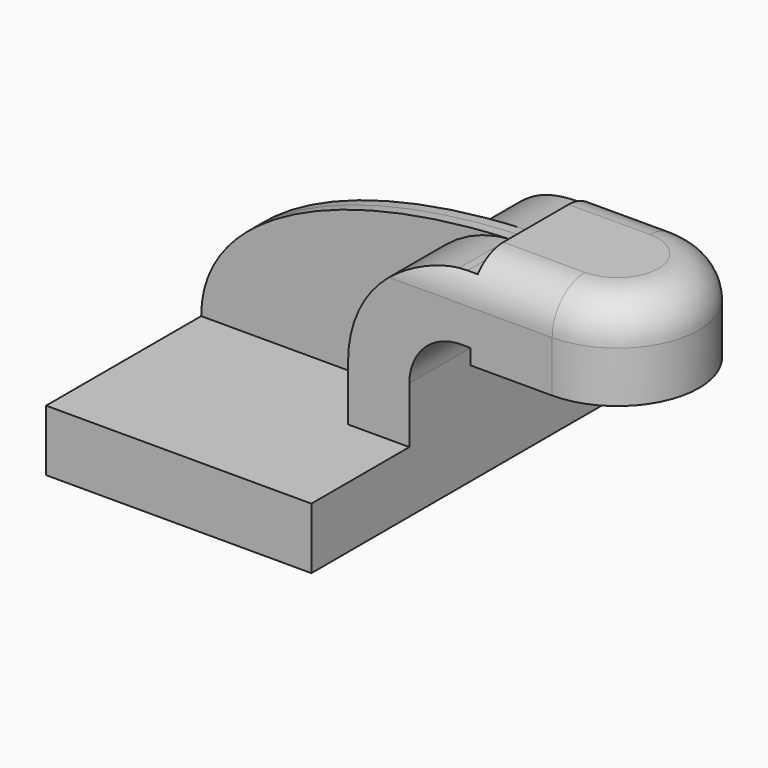
from build123d import *

# Parameters (mm, degrees)
F1_DEPTH = 63.5
F0_W     = 25.4
F0_H     = 19.05
F0_H_2   = 4.7498
F0_H_3   = 4.7752
F2_DEPTH = 25.4
F4_DEPTH = 3.175
F5_R     = 12.7


with BuildPart() as f1:
    # F0 (on Front) → F1 (new body, symmetric)
    with BuildSketch(Plane.XZ):
        Polygon((-41.275, -9.525), (41.275, -9.525), (41.275, 9.525), (22.225, 9.525), (-41.275, 9.525), align=None)
    extrude(amount=F1_DEPTH, both=True)

    # F0 (on Front) → F2 (join, symmetric)
    with BuildSketch(Plane.XZ):
        with BuildLine():
            Line((22.225, 9.525), (41.275, 9.525))
            Line((41.275, 9.525), (41.275, 27.0002))
            ThreePointArc((41.275, 27.0002), (45.9246798487, 38.2255201513), (57.15, 42.8752))
            Line((57.15, 42.8752), (60.325, 42.8752))
            Line((60.325, 42.8752), (60.325, 61.9252))
            Line((60.325, 61.9252), (57.15, 61.9252))
            add(Edge.make_bspline(
                [(54.6251217416, 61.8338132892), (55.4640803854, 61.8685780106), (56.3057470428, 61.8990488271), (57.15, 61.9252)],
                knots=[109.7820212307, 109.7820212307, 109.7820212307, 109.7820212307, 111.5045361635, 111.5045361635, 111.5045361635, 111.5045361635], degree=3))
            ThreePointArc((54.6251217416, 61.8338132892), (31.5771921939, 50.7864802033), (22.225, 27.0002))
            Line((22.225, 27.0002), (22.225, 9.525))
        make_face()
        with Locations((73.025, 52.4002)):
            Rectangle(F0_W, F0_H)
        with Locations((73.025, 64.3001)):
            Rectangle(F0_W, F0_H_2)
        with Locations((73.025, 40.4876)):
            Rectangle(F0_W, F0_H_3)
    extrude(amount=F2_DEPTH, both=True)

    # F0 (on Front) → F3 (revolve)
    with BuildSketch(Plane.XZ):
        Polygon((85.725, 61.9252), (85.725, 42.8752), (85.725, 38.1), (111.125, 38.1), (111.125, 66.675), (85.725, 66.675), align=None)
    revolve(axis=Axis((85.725, 0, 52.3875), (0, 0, 1)))

    # F0 (on Front) → F4 (join, symmetric)
    with BuildSketch(Plane.XZ):
        with BuildLine():
            add(Edge.make_bspline(
                [(-41.275, 9.525), (-41.3146686629, 39.9607514864), (1.1552946366, 59.618133583), (54.6251217416, 61.8338132892)],
                knots=[0, 0, 0, 0, 109.7820212307, 109.7820212307, 109.7820212307, 109.7820212307], degree=3))
            Line((-41.275, 9.525), (22.225, 9.525))
            Line((22.225, 9.525), (22.225, 27.0002))
            ThreePointArc((22.225, 27.0002), (31.5771921939, 50.7864802033), (54.6251217416, 61.8338132892))
        make_face()
    extrude(amount=F4_DEPTH, both=True)

    # F5
    f5_edges = [f1.edges().sort_by_distance(p)[0] for p in [
        (85.725, 25.4, 52.3875),
        (73.025, 25.4, 66.675),
        (73.025, -25.4, 66.675),
        (111.125, 0, 66.675),
    ]]
    fillet(f5_edges, radius=F5_R)


solid = f1.part
